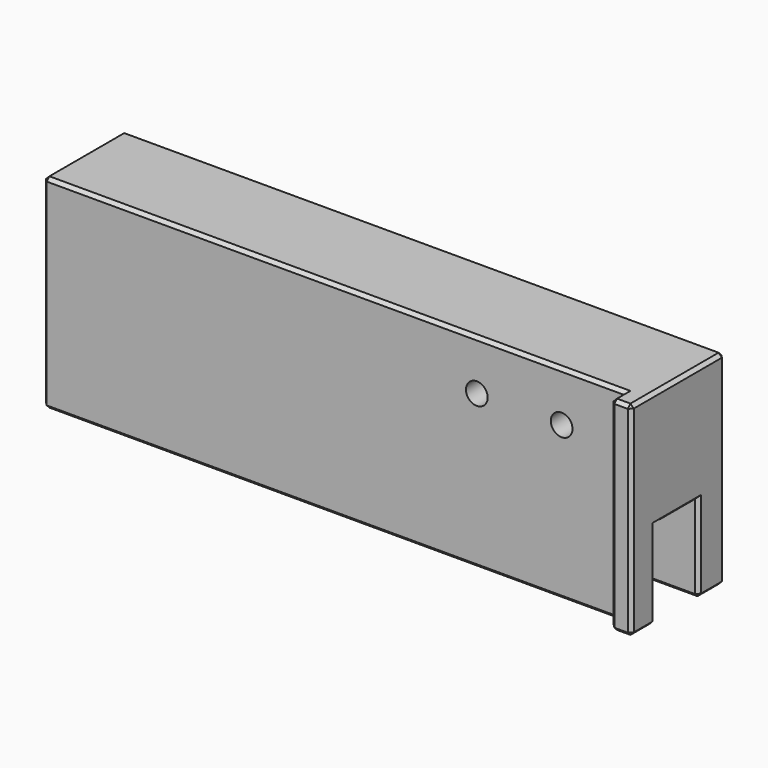
from build123d import *

# Parameters (mm, degrees)
F1_DEPTH = 90
F2_W     = 6
F2_H     = 61
F3_DEPTH = 5
F4_R     = 3.25
F5_DEPTH = 30.001
F7_DEPTH = 7
F8_SIZE  = 0.99999
F9_SIZE  = 1


# Not quite as in the source:
# - a fillet or chamfer is up to 0.001 mm smaller than in the source, because OpenCascade refuses the exact size


with BuildPart() as f1:
    # F0 (on Right) → F1 (new body, symmetric)
    with BuildSketch(Plane.YZ):
        Polygon((-6.05, 13), (8.05, 13), (8.05, -13), (17.95, -13), (17.95, 48), (-12.05, 48), (-12.05, -13), (-8.05, -13), (-8.05, 14), (-6.05, 14), align=None)
    extrude(amount=F1_DEPTH, both=True)

    # F2 (on face) → F3 (join)
    with BuildSketch(Plane.XZ.offset(12.05)):
        with Locations((87, 17.5)):
            Rectangle(F2_W, F2_H)
    extrude(amount=F3_DEPTH)

    # F4 (on face) → F5 (cut, through all)
    with BuildSketch(Plane.XZ.offset(12.05)):
        with Locations((39.8, 33)):
            Circle(F4_R)
        with Locations((65.2, 33)):
            Circle(F4_R)
    extrude(amount=-F5_DEPTH, mode=Mode.SUBTRACT)

    # F6 (on face) → F7 (cut)
    with BuildSketch(Plane(origin=(0, 17.95, 0), x_dir=(-1, 0, 0), z_dir=(0, 1, 0))):
        Polygon((-61.9668384925, 38.6), (-68.4331615075, 38.6), (-71.6663230149, 33), (-68.4331615075, 27.4), (-61.9668384925, 27.4), (-58.7336769851, 33), align=None)
        Polygon((-36.5668384925, 38.6), (-43.0331615075, 38.6), (-46.2663230149, 33), (-43.0331615075, 27.4), (-36.5668384925, 27.4), (-33.3336769851, 33), align=None)
    extrude(amount=-F7_DEPTH, mode=Mode.SUBTRACT)

    # F8 (size 1 in the source; OpenCascade refuses exactly that, so slightly less here)
    f8_edges = [f1.edges().sort_by_distance(p)[0] for p in [
        (0, -6.05, 13),
    ]]
    chamfer(f8_edges, length=F8_SIZE)

    # F9
    f9_edges = [f1.edges().sort_by_distance(p)[0] for p in [
        (0, -8.05, -13),
        (0, 8.05, -13),
        (0, 17.95, -13),
        (-90, 13, -13),
        (-90, 8.05, 0),
        (90, 13, -13),
        (-3, -12.05, -13),
        (-90, -10.05, -13),
        (84, -14.55, -13),
        (90, -12.55, -13),
        (87, -17.05, -13),
        (-90, -12.05, 17.5),
        (-90, 17.95, 17.5),
        (-90, -8.05, 0.5),
        (90, 8.05, 0),
        (90, -8.05, 0.5),
        (90, 1.499995, 13),
        (-90, 1.499995, 13),
        (90, 0.45, 48),
        (90, 17.95, 17.5),
        (0, 17.95, 48),
        (-3, -12.05, 48),
        (-90, 2.95, 48),
        (87, -17.05, 48),
        (84, -14.55, 48),
        (90, -17.05, 17.5),
        (84, -17.05, 17.5),
    ]]
    chamfer(f9_edges, length=F9_SIZE)


solid = f1.part
